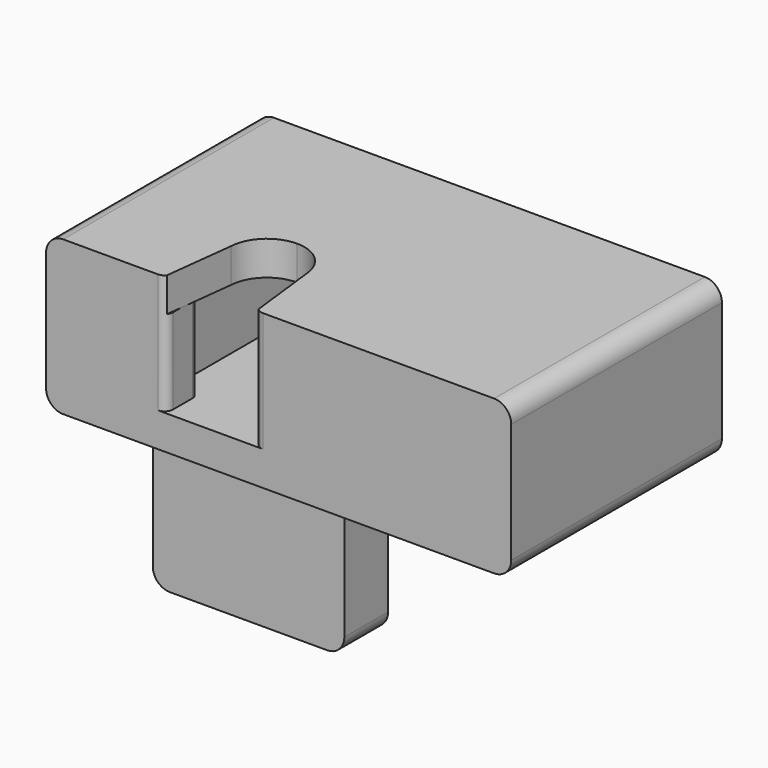
from build123d import *

# Parameters (mm, degrees)
F0_W         = 5.6
F0_H         = 4.5
F0_W_2       = 3.97
F0_H_2       = 2.5
F1_DEPTH     = 7.7
F2_W         = 5.6
F2_H         = 1.6
F3_DEPTH     = 4.5
F4_W         = 1.2
F4_H         = 2.5
F5_DEPTH     = 0.7
F8_DEPTH     = 6
F10_DEPTH    = 1
F12_DEPTH    = 2
F13_R        = 0.5
F14_T1_DEPTH = 4
F14_T3_DEPTH = 2.5


# Not quite as in the source:
# - a fillet or chamfer that OpenCascade refuses, or shapes differently, is made with other operations: its cross-section is extruded or revolved along the edge and cut away or added
# - a pattern or mirror of a feature is missing from the dataset's text; its kind, count and spacing are read off the source's solid


with BuildPart() as f1:
    # F0 (on Front) → F1 (new body)
    with BuildSketch(Plane.XZ):
        Rectangle(F0_W, F0_H)
        Rectangle(F0_W_2, F0_H_2, mode=Mode.SUBTRACT)
    extrude(amount=F1_DEPTH)

    # F2 (on face) → F3 (join)
    with BuildSketch(Plane(origin=(0, 0, -2.25), x_dir=(1, 0, 0), z_dir=(0, 0, -1))):
        with Locations((0, 5.5)):
            Rectangle(F2_W, F2_H)
    extrude(amount=F3_DEPTH)

    # F4 (on face) → F5 (join)
    with BuildSketch(Plane.YZ.offset(-1.985)):
        with Locations((-7.1, 0)):
            Rectangle(F4_W, F4_H)
    f5 = extrude(amount=F5_DEPTH)

    # F5_copies: F5 across plane
    add(f5.mirror(Plane(origin=(0, 0, 0), x_dir=(0, 0, 1), z_dir=(1, 0, 0))))

    # F7 (on face) → F8 (join)
    with BuildSketch(Plane.YZ.offset(2.8)):
        Polygon((0, 2.25), (-7.7, 2.25), (-7.7, -2.25), (-6.3, -2.25), (-4.7, -2.25), (0, -2.25), align=None)
    extrude(amount=F8_DEPTH)

    # F9 (on face) → F10 (cut)
    with BuildSketch(Plane.XY.offset(2.25)):
        with BuildLine():
            ThreePointArc((-1.0984344714, -5.5712931935), (-0.0293434956, -6.7295678482), (1.1, -5.6299593))
            ThreePointArc((1.1, -5.6299593), (1.0996085482, -5.6006158044), (1.0984344714, -5.5712931935))
            ThreePointArc((1.0984344714, -5.5712931935), (0.7567916764, -4.8316696542), (0, -4.5299593))
            ThreePointArc((0, -4.5299593), (-0.7567916764, -4.8316696542), (-1.0984344714, -5.5712931935))
        make_face()
        with BuildLine():
            ThreePointArc((1.0984344714, -5.5712931935), (1.0996085482, -5.6006158044), (1.1, -5.6299593))
            ThreePointArc((1.1, -5.6299593), (-0.0293434956, -6.7295678482), (-1.0984344714, -5.5712931935))
            Line((-1.0984344714, -5.5712931935), (-1.35, -7.7))
            Line((-1.35, -7.7), (1.35, -7.7))
            Line((1.35, -7.7), (1.0984344714, -5.5712931935))
        make_face()
    extrude(amount=-F10_DEPTH, mode=Mode.SUBTRACT)

    # F11 (on face) → F12 (join)
    with BuildSketch(Plane(origin=(-2.8, 0, 0), x_dir=(0, -1, 0), z_dir=(-1, 0, 0))):
        Polygon((7.7, -2.25), (7.7, 2.25), (0, 2.25), (0, -2.25), (4.7, -2.25), (6.3, -2.25), align=None)
    extrude(amount=F12_DEPTH)

    # F13
    f13_edges = [f1.edges().sort_by_distance(p)[0] for p in [
        (8.8, -3.85, -2.25),
        (8.8, -3.85, 2.25),
        (2.8, -5.5, -6.75),
        (-4.8, -3.85, 2.25),
        (-4.8, -3.85, -2.25),
        (-2.8, -5.5, -6.75),
    ]]
    fillet(f13_edges, radius=F13_R)

    # F14: fillet of radius 0.25 on 4 edges, made by hand

    # F14_s2 → F14_t1 (cut)
    with BuildSketch(Plane.XY.offset(-1.25)):
        with BuildLine():
            ThreePointArc((-1.535, -7.7), (-1.3582233047, -7.6267766953), (-1.285, -7.45))
            Line((-1.285, -7.45), (-1.28, -7.45))
            Line((-1.28, -7.45), (-1.28, -7.705))
            Line((-1.28, -7.705), (-1.535, -7.705))
            Line((-1.535, -7.705), (-1.535, -7.7))
        make_face()
        with BuildLine():
            ThreePointArc((1.535, -7.7), (1.3582233047, -7.6267766953), (1.285, -7.45))
            Line((1.285, -7.45), (1.28, -7.45))
            Line((1.28, -7.45), (1.28, -7.705))
            Line((1.28, -7.705), (1.535, -7.705))
            Line((1.535, -7.705), (1.535, -7.7))
        make_face()
    extrude(amount=F14_T1_DEPTH, mode=Mode.SUBTRACT)

    # F14_s4 → F14_t3 (cut)
    with BuildSketch(Plane.XY.offset(-1.25)):
        with BuildLine():
            ThreePointArc((-1.285, -6.75), (-1.3582233047, -6.5732233047), (-1.535, -6.5))
            Line((-1.535, -6.5), (-1.535, -6.495))
            Line((-1.535, -6.495), (-1.28, -6.495))
            Line((-1.28, -6.495), (-1.28, -6.75))
            Line((-1.28, -6.75), (-1.285, -6.75))
        make_face()
        with BuildLine():
            ThreePointArc((1.285, -6.75), (1.3582233047, -6.5732233047), (1.535, -6.5))
            Line((1.535, -6.5), (1.535, -6.495))
            Line((1.535, -6.495), (1.28, -6.495))
            Line((1.28, -6.495), (1.28, -6.75))
            Line((1.28, -6.75), (1.285, -6.75))
        make_face()
    extrude(amount=F14_T3_DEPTH, mode=Mode.SUBTRACT)


solid = f1.part
